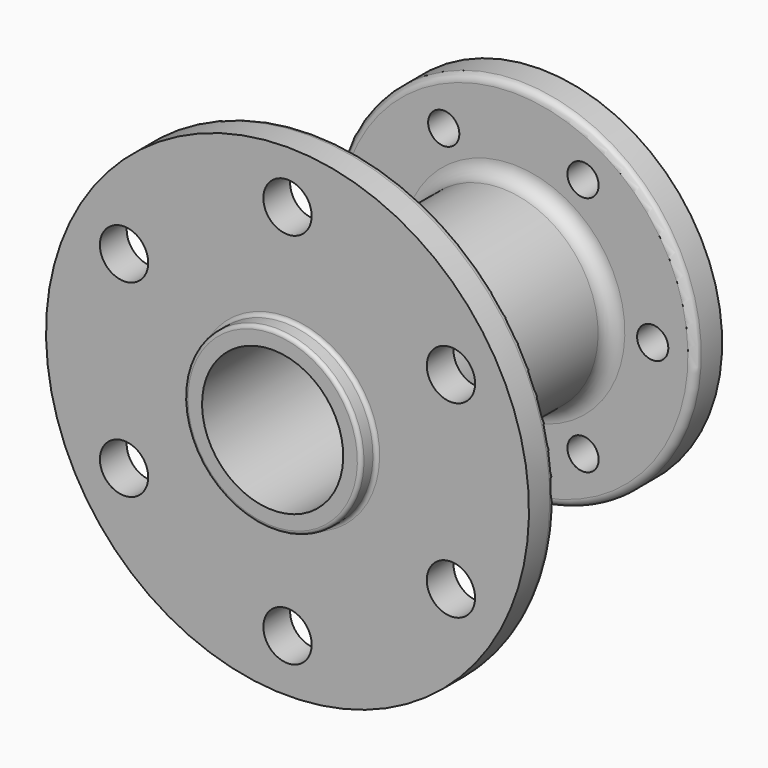
from build123d import *

# Parameters (mm, degrees)
F3_D            = 8.4
F3_DEPTH        = 15
F3_TIP          = 2.5236145999
F3_COPIES_COUNT = 6
F4_R            = 6.5
F5_DEPTH        = 18
F5_COPIES_COUNT = 6


# Not quite as in the source:
# - a pattern or mirror of a feature is missing from the dataset's text; its kind, count and spacing are read off the source's solid


with BuildPart() as f1:
    # F0 (on Right) → F1 (revolve)
    with BuildSketch(Plane.YZ):
        with BuildLine():
            Line((89, 28), (85, 28))
            Line((85, 28), (85, 49))
            Line((85, 49), (78, 49))
            ThreePointArc((78, 49), (76.5857864376, 48.4142135624), (76, 47))
            Line((76, 47), (76, 30))
            ThreePointArc((76, 30), (74.8284271247, 27.1715728753), (72, 26))
            Line((72, 26), (14, 26))
            ThreePointArc((14, 26), (10.4644660941, 27.4644660941), (9, 31))
            Line((9, 31), (9, 63))
            ThreePointArc((9, 63), (8.4142135624, 64.4142135624), (7, 65))
            Line((7, 65), (0, 65))
            Line((0, 65), (0, 24.8))
            ThreePointArc((0, 24.8), (-0.2928932188, 24.0928932188), (-1, 23.8))
            Line((-1, 23.8), (-4, 23.8))
            ThreePointArc((-4, 23.8), (-4.7071067812, 23.5071067812), (-5, 22.8))
            Line((-5, 22.8), (-5, 19))
            Line((-5, 19), (0, 19))
            Line((0, 19), (85, 19))
            Line((85, 19), (90, 19))
            Line((90, 19), (90, 27))
            ThreePointArc((90, 27), (89.7071067812, 27.7071067812), (89, 28))
        make_face()
    revolve(axis=Axis((0, 2.4354029447, 0), (0, 1, 0)))

    # F3
    with Locations(Plane(origin=(0, 85, 0), x_dir=(-1, 0, 0), z_dir=(0, 1, 0))):
        with Locations((37.5, 0)):
            f3 = Hole(F3_D / 2, depth=F3_DEPTH)
            with Locations((0, 0, -(F3_DEPTH + F3_TIP / 2))):  # 118° drill point
                Cone(0, F3_D / 2, F3_TIP, mode=Mode.SUBTRACT)

    # F3_copies: F3 ×6 about axis
    f3_copies_axis = Axis((0, 0, 0), (0, 1, 0))
    for i in range(1, F3_COPIES_COUNT):
        add(f3.rotate(f3_copies_axis, i * 360 / F3_COPIES_COUNT), mode=Mode.SUBTRACT)

    # F4 (on Front) → F5 (cut)
    with BuildSketch(Plane.XZ):
        with Locations((0, 50.8)):
            Circle(F4_R)
    f5 = extrude(amount=-F5_DEPTH, mode=Mode.SUBTRACT)

    # F5_copies: F5 ×6 about axis
    f5_copies_axis = Axis((0, 0, 0), (0, 1, 0))
    for i in range(1, F5_COPIES_COUNT):
        add(f5.rotate(f5_copies_axis, i * 360 / F5_COPIES_COUNT), mode=Mode.SUBTRACT)


solid = f1.part
